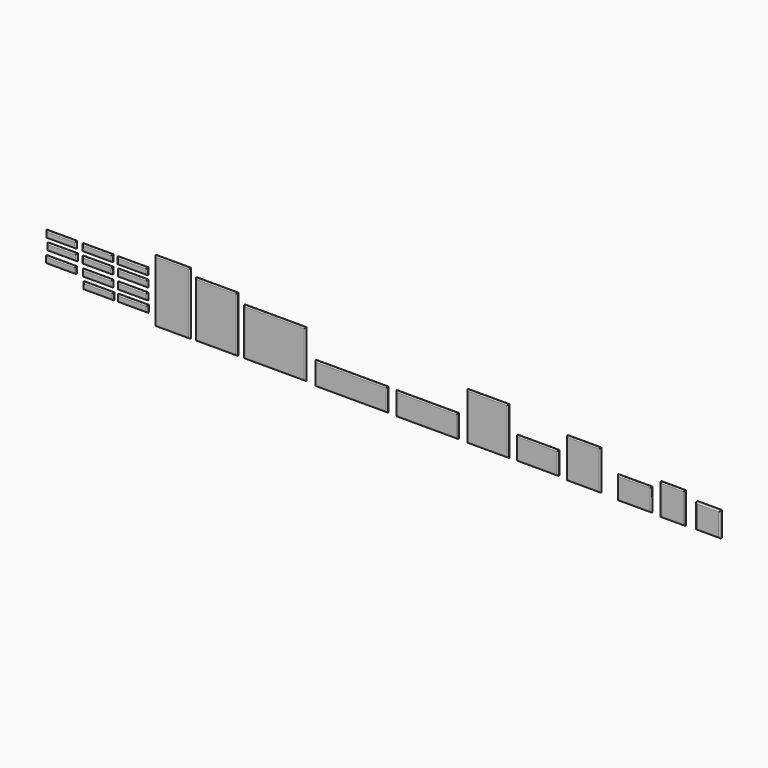
from build123d import *

# Parameters (mm, degrees)
F0_W           = 123
F0_H           = 28
F1_DEPTH       = 10
F2_T           = -2.5
F2_2_T         = -2.5
F2_3_T         = -2.5
F2_4_T         = -2.5
F2_5_T         = -2.5
F2_6_T         = -2.5
F2_7_T         = -2.5
F2_8_T         = -2.5
F2_9_T         = -2.5
F2_10_T        = -2.5
F2_11_T        = -2.5
F3_W           = 144
F3_H           = 255
F4_DEPTH       = 10
F3_W_2         = 170
F3_H_2         = 227
F3_W_3         = 253
F3_H_3         = 193
F3_W_4         = 296
F3_H_4         = 93
F3_W_5         = 139
F3_H_5         = 162
F3_W_6         = 100
F3_H_6         = 128
F3_H_7         = 100
F5_T           = -2.5
F5_2_T         = -2.5
F5_3_T         = -2.5
F5_4_T         = -2.5
F5_5_T         = -2.5
F5_6_T         = -2.5
F5_7_T         = -2.5
F5_8_T         = -2.5
F5_9_T         = -2.5
F5_10_T        = -2.5
F5_11_T        = -2.5
F6_T1_DEPTH    = 169
F6_T3_DEPTH    = 280
F6_2_T1_DEPTH  = 252
F6_2_T3_DEPTH  = 195
F6_3_T1_DEPTH  = 278
F6_3_T3_DEPTH  = 218
F6_4_T1_DEPTH  = 118
F6_4_T3_DEPTH  = 321
F6_5_T1_DEPTH  = 278
F6_5_T3_DEPTH  = 118
F6_6_T1_DEPTH  = 195
F6_6_T3_DEPTH  = 218
F6_7_T1_DEPTH  = 195
F6_7_T3_DEPTH  = 118
F6_8_T1_DEPTH  = 164
F6_8_T3_DEPTH  = 187
F6_9_T1_DEPTH  = 164
F6_9_T3_DEPTH  = 118
F6_10_T1_DEPTH = 125
F6_10_T3_DEPTH = 153
F6_11_T1_DEPTH = 125
F6_11_T3_DEPTH = 125
F6_12_T1_DEPTH = 53
F6_12_T3_DEPTH = 148
F6_13_T1_DEPTH = 148
F6_13_T3_DEPTH = 53
F6_14_T1_DEPTH = 148
F6_14_T3_DEPTH = 53
F6_15_T1_DEPTH = 148
F6_15_T3_DEPTH = 53
F6_16_T1_DEPTH = 53
F6_16_T3_DEPTH = 148
F6_17_T1_DEPTH = 53
F6_17_T3_DEPTH = 148
F6_18_T1_DEPTH = 53
F6_18_T3_DEPTH = 148
F6_19_T1_DEPTH = 148
F6_19_T3_DEPTH = 53
F6_20_T1_DEPTH = 53
F6_20_T3_DEPTH = 148
F6_21_T1_DEPTH = 148
F6_21_T3_DEPTH = 53
F6_22_T1_DEPTH = 53
F6_22_T3_DEPTH = 148


# Not quite as in the source:
# - a fillet or chamfer that OpenCascade refuses, or shapes differently, is made with other operations: its cross-section is extruded or revolved along the edge and cut away or added


with BuildPart() as f1:
    # F0 (on Front) → F1 (new body)
    with BuildSketch(Plane.XZ):
        with Locations((-123.9206232131, 65.0202791235)):
            Rectangle(F0_W, F0_H)
    extrude(amount=F1_DEPTH)

    # F2
    f2_openings = [f1.faces().sort_by_distance(p)[0] for p in [
        (-123.920623, -5, 51.020279),
    ]]
    offset(amount=F2_T, openings=f2_openings)

    # F6#12: fillet of radius 5 on 8 edges, made by hand

    # F6_12_s2 → F6_12_t1 (cut)
    with BuildSketch(Plane.XY.offset(38.5202791235)):
        with BuildLine():
            ThreePointArc((-185.4206232131, -5), (-183.956157119, -8.5355339059), (-180.4206232131, -10))
            Line((-180.4206232131, -10), (-185.4206232131, -10))
            Line((-185.4206232131, -10), (-185.4206232131, -5))
        make_face()
        with BuildLine():
            ThreePointArc((-62.4206232131, -5), (-63.8850893071, -8.5355339059), (-67.4206232131, -10))
            Line((-67.4206232131, -10), (-62.4206232131, -10))
            Line((-62.4206232131, -10), (-62.4206232131, -5))
        make_face()
        with BuildLine():
            ThreePointArc((-185.4206232131, -5), (-183.956157119, -1.4644660941), (-180.4206232131, 0))
            Line((-180.4206232131, 0), (-185.4206232131, 0))
            Line((-185.4206232131, 0), (-185.4206232131, -5))
        make_face()
        with BuildLine():
            ThreePointArc((-62.4206232131, -5), (-63.8850893071, -1.4644660941), (-67.4206232131, 0))
            Line((-67.4206232131, 0), (-62.4206232131, 0))
            Line((-62.4206232131, 0), (-62.4206232131, -5))
        make_face()
    extrude(amount=F6_12_T1_DEPTH, mode=Mode.SUBTRACT)

    # F6_12_s4 → F6_12_t3 (cut)
    with BuildSketch(Plane.YZ.offset(-197.9206232131)):
        with BuildLine():
            ThreePointArc((-10, 56.0202791235), (-8.5355339059, 52.4847452176), (-5, 51.0202791235))
            Line((-5, 51.0202791235), (-10, 51.0202791235))
            Line((-10, 51.0202791235), (-10, 56.0202791235))
        make_face()
        with BuildLine():
            ThreePointArc((-5, 79.0202791235), (-8.5355339059, 77.5558130295), (-10, 74.0202791235))
            Line((-10, 74.0202791235), (-10, 79.0202791235))
            Line((-10, 79.0202791235), (-5, 79.0202791235))
        make_face()
        with BuildLine():
            ThreePointArc((0, 56.0202791235), (-1.4644660941, 52.4847452176), (-5, 51.0202791235))
            Line((-5, 51.0202791235), (0, 51.0202791235))
            Line((0, 51.0202791235), (0, 56.0202791235))
        make_face()
        with BuildLine():
            ThreePointArc((-5, 79.0202791235), (-1.4644660941, 77.5558130295), (0, 74.0202791235))
            Line((0, 74.0202791235), (0, 79.0202791235))
            Line((0, 79.0202791235), (-5, 79.0202791235))
        make_face()
    extrude(amount=F6_12_T3_DEPTH, mode=Mode.SUBTRACT)


with BuildPart() as f1b:
    # F0 (on Front) → F1, piece 2 (new body)
    with BuildSketch(Plane.XZ):
        with Locations((-123.1104342043, -25.217052117)):
            Rectangle(F0_W, F0_H)
    extrude(amount=F1_DEPTH)

    # F2#11
    f2_11_openings = [f1b.faces().sort_by_distance(p)[0] for p in [
        (-123.110434, -5, -39.217052),
    ]]
    offset(amount=F2_11_T, openings=f2_11_openings)

    # F6#16: fillet of radius 5 on 8 edges, made by hand

    # F6_16_s2 → F6_16_t1 (cut)
    with BuildSketch(Plane.XY.offset(-51.717052117)):
        with BuildLine():
            ThreePointArc((-61.6104342043, -5), (-63.0749002984, -8.5355339059), (-66.6104342043, -10))
            Line((-66.6104342043, -10), (-61.6104342043, -10))
            Line((-61.6104342043, -10), (-61.6104342043, -5))
        make_face()
        with BuildLine():
            ThreePointArc((-184.6104342043, -5), (-183.1459681103, -8.5355339059), (-179.6104342043, -10))
            Line((-179.6104342043, -10), (-184.6104342043, -10))
            Line((-184.6104342043, -10), (-184.6104342043, -5))
        make_face()
        with BuildLine():
            ThreePointArc((-61.6104342043, -5), (-63.0749002984, -1.4644660941), (-66.6104342043, 0))
            Line((-66.6104342043, 0), (-61.6104342043, 0))
            Line((-61.6104342043, 0), (-61.6104342043, -5))
        make_face()
        with BuildLine():
            ThreePointArc((-184.6104342043, -5), (-183.1459681103, -1.4644660941), (-179.6104342043, 0))
            Line((-179.6104342043, 0), (-184.6104342043, 0))
            Line((-184.6104342043, 0), (-184.6104342043, -5))
        make_face()
    extrude(amount=F6_16_T1_DEPTH, mode=Mode.SUBTRACT)

    # F6_16_s4 → F6_16_t3 (cut)
    with BuildSketch(Plane.YZ.offset(-197.1104342043)):
        with BuildLine():
            ThreePointArc((-5, -11.217052117), (-8.5355339059, -12.6815182111), (-10, -16.217052117))
            Line((-10, -16.217052117), (-10, -11.217052117))
            Line((-10, -11.217052117), (-5, -11.217052117))
        make_face()
        with BuildLine():
            ThreePointArc((-10, -34.217052117), (-8.5355339059, -37.7525860229), (-5, -39.217052117))
            Line((-5, -39.217052117), (-10, -39.217052117))
            Line((-10, -39.217052117), (-10, -34.217052117))
        make_face()
        with BuildLine():
            ThreePointArc((-5, -11.217052117), (-1.4644660941, -12.6815182111), (0, -16.217052117))
            Line((0, -16.217052117), (0, -11.217052117))
            Line((0, -11.217052117), (-5, -11.217052117))
        make_face()
        with BuildLine():
            ThreePointArc((0, -34.217052117), (-1.4644660941, -37.7525860229), (-5, -39.217052117))
            Line((-5, -39.217052117), (0, -39.217052117))
            Line((0, -39.217052117), (0, -34.217052117))
        make_face()
    extrude(amount=F6_16_T3_DEPTH, mode=Mode.SUBTRACT)


with BuildPart() as f1c:
    # F0 (on Front) → F1, piece 3 (new body)
    with BuildSketch(Plane.XZ):
        with Locations((-122.2762821019, -69.5036254227)):
            Rectangle(F0_W, F0_H)
    extrude(amount=F1_DEPTH)

    # F2#10
    f2_10_openings = [f1c.faces().sort_by_distance(p)[0] for p in [
        (-122.276282, -5, -83.503625),
    ]]
    offset(amount=F2_10_T, openings=f2_10_openings)

    # F6#15: fillet of radius 5 on 8 edges, made by hand

    # F6_15_s2 → F6_15_t1 (cut)
    with BuildSketch(Plane.YZ.offset(-196.2762821019)):
        with BuildLine():
            ThreePointArc((-5, -55.5036254227), (-8.5355339059, -56.9680915168), (-10, -60.5036254227))
            Line((-10, -60.5036254227), (-10, -55.5036254227))
            Line((-10, -55.5036254227), (-5, -55.5036254227))
        make_face()
        with BuildLine():
            ThreePointArc((-10, -78.5036254227), (-8.5355339059, -82.0391593286), (-5, -83.5036254227))
            Line((-5, -83.5036254227), (-10, -83.5036254227))
            Line((-10, -83.5036254227), (-10, -78.5036254227))
        make_face()
        with BuildLine():
            ThreePointArc((-5, -55.5036254227), (-1.4644660941, -56.9680915168), (0, -60.5036254227))
            Line((0, -60.5036254227), (0, -55.5036254227))
            Line((0, -55.5036254227), (-5, -55.5036254227))
        make_face()
        with BuildLine():
            ThreePointArc((0, -78.5036254227), (-1.4644660941, -82.0391593286), (-5, -83.5036254227))
            Line((-5, -83.5036254227), (0, -83.5036254227))
            Line((0, -83.5036254227), (0, -78.5036254227))
        make_face()
    extrude(amount=F6_15_T1_DEPTH, mode=Mode.SUBTRACT)

    # F6_15_s4 → F6_15_t3 (cut)
    with BuildSketch(Plane.XY.offset(-96.0036254227)):
        with BuildLine():
            ThreePointArc((-183.7762821019, -5), (-182.3118160078, -8.5355339059), (-178.7762821019, -10))
            Line((-178.7762821019, -10), (-183.7762821019, -10))
            Line((-183.7762821019, -10), (-183.7762821019, -5))
        make_face()
        with BuildLine():
            ThreePointArc((-60.7762821019, -5), (-62.2407481959, -8.5355339059), (-65.7762821019, -10))
            Line((-65.7762821019, -10), (-60.7762821019, -10))
            Line((-60.7762821019, -10), (-60.7762821019, -5))
        make_face()
        with BuildLine():
            ThreePointArc((-183.7762821019, -5), (-182.3118160078, -1.4644660941), (-178.7762821019, 0))
            Line((-178.7762821019, 0), (-183.7762821019, 0))
            Line((-183.7762821019, 0), (-183.7762821019, -5))
        make_face()
        with BuildLine():
            ThreePointArc((-60.7762821019, -5), (-62.2407481959, -1.4644660941), (-65.7762821019, 0))
            Line((-65.7762821019, 0), (-60.7762821019, 0))
            Line((-60.7762821019, 0), (-60.7762821019, -5))
        make_face()
    extrude(amount=F6_15_T3_DEPTH, mode=Mode.SUBTRACT)


with BuildPart() as f1d:
    # F0 (on Front) → F1, piece 4 (new body)
    with BuildSketch(Plane.XZ):
        with Locations((-267.2222574949, 65.6239078045)):
            Rectangle(F0_W, F0_H)
    extrude(amount=F1_DEPTH)

    # F2#4
    f2_4_openings = [f1d.faces().sort_by_distance(p)[0] for p in [
        (-267.222257, -5, 51.623908),
    ]]
    offset(amount=F2_4_T, openings=f2_4_openings)

    # F6#14: fillet of radius 5 on 8 edges, made by hand

    # F6_14_s2 → F6_14_t1 (cut)
    with BuildSketch(Plane.YZ.offset(-341.2222574949)):
        with BuildLine():
            ThreePointArc((-5, 79.6239078045), (-8.5355339059, 78.1594417104), (-10, 74.6239078045))
            Line((-10, 74.6239078045), (-10, 79.6239078045))
            Line((-10, 79.6239078045), (-5, 79.6239078045))
        make_face()
        with BuildLine():
            ThreePointArc((-10, 56.6239078045), (-8.5355339059, 53.0883738986), (-5, 51.6239078045))
            Line((-5, 51.6239078045), (-10, 51.6239078045))
            Line((-10, 51.6239078045), (-10, 56.6239078045))
        make_face()
        with BuildLine():
            ThreePointArc((-5, 79.6239078045), (-1.4644660941, 78.1594417104), (0, 74.6239078045))
            Line((0, 74.6239078045), (0, 79.6239078045))
            Line((0, 79.6239078045), (-5, 79.6239078045))
        make_face()
        with BuildLine():
            ThreePointArc((0, 56.6239078045), (-1.4644660941, 53.0883738986), (-5, 51.6239078045))
            Line((-5, 51.6239078045), (0, 51.6239078045))
            Line((0, 51.6239078045), (0, 56.6239078045))
        make_face()
    extrude(amount=F6_14_T1_DEPTH, mode=Mode.SUBTRACT)

    # F6_14_s4 → F6_14_t3 (cut)
    with BuildSketch(Plane.XY.offset(39.1239078045)):
        with BuildLine():
            ThreePointArc((-328.7222574949, -5), (-327.2577914009, -8.5355339059), (-323.7222574949, -10))
            Line((-323.7222574949, -10), (-328.7222574949, -10))
            Line((-328.7222574949, -10), (-328.7222574949, -5))
        make_face()
        with BuildLine():
            ThreePointArc((-205.7222574949, -5), (-207.186723589, -8.5355339059), (-210.7222574949, -10))
            Line((-210.7222574949, -10), (-205.7222574949, -10))
            Line((-205.7222574949, -10), (-205.7222574949, -5))
        make_face()
        with BuildLine():
            ThreePointArc((-328.7222574949, -5), (-327.2577914009, -1.4644660941), (-323.7222574949, 0))
            Line((-323.7222574949, 0), (-328.7222574949, 0))
            Line((-328.7222574949, 0), (-328.7222574949, -5))
        make_face()
        with BuildLine():
            ThreePointArc((-205.7222574949, -5), (-207.186723589, -1.4644660941), (-210.7222574949, 0))
            Line((-210.7222574949, 0), (-205.7222574949, 0))
            Line((-205.7222574949, 0), (-205.7222574949, -5))
        make_face()
    extrude(amount=F6_14_T3_DEPTH, mode=Mode.SUBTRACT)


with BuildPart() as f1e:
    # F0 (on Front) → F1, piece 5 (new body)
    with BuildSketch(Plane.XZ):
        with Locations((-123.2876462638, 21.4466401041)):
            Rectangle(F0_W, F0_H)
    extrude(amount=F1_DEPTH)

    # F2#2
    f2_2_openings = [f1e.faces().sort_by_distance(p)[0] for p in [
        (-123.287646, -5, 7.44664),
    ]]
    offset(amount=F2_2_T, openings=f2_2_openings)

    # F6#13: fillet of radius 5 on 8 edges, made by hand

    # F6_13_s2 → F6_13_t1 (cut)
    with BuildSketch(Plane.YZ.offset(-197.2876462638)):
        with BuildLine():
            ThreePointArc((-5, 35.4466401041), (-8.5355339059, 33.98217401), (-10, 30.4466401041))
            Line((-10, 30.4466401041), (-10, 35.4466401041))
            Line((-10, 35.4466401041), (-5, 35.4466401041))
        make_face()
        with BuildLine():
            ThreePointArc((-10, 12.4466401041), (-8.5355339059, 8.9111061981), (-5, 7.4466401041))
            Line((-5, 7.4466401041), (-10, 7.4466401041))
            Line((-10, 7.4466401041), (-10, 12.4466401041))
        make_face()
        with BuildLine():
            ThreePointArc((-5, 35.4466401041), (-1.4644660941, 33.98217401), (0, 30.4466401041))
            Line((0, 30.4466401041), (0, 35.4466401041))
            Line((0, 35.4466401041), (-5, 35.4466401041))
        make_face()
        with BuildLine():
            ThreePointArc((0, 12.4466401041), (-1.4644660941, 8.9111061981), (-5, 7.4466401041))
            Line((-5, 7.4466401041), (0, 7.4466401041))
            Line((0, 7.4466401041), (0, 12.4466401041))
        make_face()
    extrude(amount=F6_13_T1_DEPTH, mode=Mode.SUBTRACT)

    # F6_13_s4 → F6_13_t3 (cut)
    with BuildSketch(Plane.XY.offset(-5.0533598959)):
        with BuildLine():
            ThreePointArc((-184.7876462638, -5), (-183.3231801698, -8.5355339059), (-179.7876462638, -10))
            Line((-179.7876462638, -10), (-184.7876462638, -10))
            Line((-184.7876462638, -10), (-184.7876462638, -5))
        make_face()
        with BuildLine():
            ThreePointArc((-61.7876462638, -5), (-63.2521123579, -8.5355339059), (-66.7876462638, -10))
            Line((-66.7876462638, -10), (-61.7876462638, -10))
            Line((-61.7876462638, -10), (-61.7876462638, -5))
        make_face()
        with BuildLine():
            ThreePointArc((-184.7876462638, -5), (-183.3231801698, -1.4644660941), (-179.7876462638, 0))
            Line((-179.7876462638, 0), (-184.7876462638, 0))
            Line((-184.7876462638, 0), (-184.7876462638, -5))
        make_face()
        with BuildLine():
            ThreePointArc((-61.7876462638, -5), (-63.2521123579, -1.4644660941), (-66.7876462638, 0))
            Line((-66.7876462638, 0), (-61.7876462638, 0))
            Line((-61.7876462638, 0), (-61.7876462638, -5))
        make_face()
    extrude(amount=F6_13_T3_DEPTH, mode=Mode.SUBTRACT)


with BuildPart() as f1f:
    # F0 (on Front) → F1, piece 6 (new body)
    with BuildSketch(Plane.XZ):
        with Locations((-267.200274229, 20.9451825023)):
            Rectangle(F0_W, F0_H)
    extrude(amount=F1_DEPTH)

    # F2#9
    f2_9_openings = [f1f.faces().sort_by_distance(p)[0] for p in [
        (-267.200274, -5, 6.945183),
    ]]
    offset(amount=F2_9_T, openings=f2_9_openings)

    # F6#17: fillet of radius 5 on 8 edges, made by hand

    # F6_17_s2 → F6_17_t1 (cut)
    with BuildSketch(Plane.XY.offset(-5.5548174977)):
        with BuildLine():
            ThreePointArc((-205.700274229, -5), (-207.1647403231, -8.5355339059), (-210.700274229, -10))
            Line((-210.700274229, -10), (-205.700274229, -10))
            Line((-205.700274229, -10), (-205.700274229, -5))
        make_face()
        with BuildLine():
            ThreePointArc((-328.700274229, -5), (-327.235808135, -8.5355339059), (-323.700274229, -10))
            Line((-323.700274229, -10), (-328.700274229, -10))
            Line((-328.700274229, -10), (-328.700274229, -5))
        make_face()
        with BuildLine():
            ThreePointArc((-205.700274229, -5), (-207.1647403231, -1.4644660941), (-210.700274229, 0))
            Line((-210.700274229, 0), (-205.700274229, 0))
            Line((-205.700274229, 0), (-205.700274229, -5))
        make_face()
        with BuildLine():
            ThreePointArc((-328.700274229, -5), (-327.235808135, -1.4644660941), (-323.700274229, 0))
            Line((-323.700274229, 0), (-328.700274229, 0))
            Line((-328.700274229, 0), (-328.700274229, -5))
        make_face()
    extrude(amount=F6_17_T1_DEPTH, mode=Mode.SUBTRACT)

    # F6_17_s4 → F6_17_t3 (cut)
    with BuildSketch(Plane.YZ.offset(-341.200274229)):
        with BuildLine():
            ThreePointArc((-5, 34.9451825023), (-8.5355339059, 33.4807164082), (-10, 29.9451825023))
            Line((-10, 29.9451825023), (-10, 34.9451825023))
            Line((-10, 34.9451825023), (-5, 34.9451825023))
        make_face()
        with BuildLine():
            ThreePointArc((-10, 11.9451825023), (-8.5355339059, 8.4096485963), (-5, 6.9451825023))
            Line((-5, 6.9451825023), (-10, 6.9451825023))
            Line((-10, 6.9451825023), (-10, 11.9451825023))
        make_face()
        with BuildLine():
            ThreePointArc((-5, 34.9451825023), (-1.4644660941, 33.4807164082), (0, 29.9451825023))
            Line((0, 29.9451825023), (0, 34.9451825023))
            Line((0, 34.9451825023), (-5, 34.9451825023))
        make_face()
        with BuildLine():
            ThreePointArc((0, 11.9451825023), (-1.4644660941, 8.4096485963), (-5, 6.9451825023))
            Line((-5, 6.9451825023), (0, 6.9451825023))
            Line((0, 6.9451825023), (0, 11.9451825023))
        make_face()
    extrude(amount=F6_17_T3_DEPTH, mode=Mode.SUBTRACT)


with BuildPart() as f1g:
    # F0 (on Front) → F1, piece 7 (new body)
    with BuildSketch(Plane.XZ):
        with Locations((-415.5285229683, 65.9489542842)):
            Rectangle(F0_W, F0_H)
    extrude(amount=F1_DEPTH)

    # F2#5
    f2_5_openings = [f1g.faces().sort_by_distance(p)[0] for p in [
        (-415.528523, -5, 51.948954),
    ]]
    offset(amount=F2_5_T, openings=f2_5_openings)

    # F6#19: fillet of radius 5 on 8 edges, made by hand

    # F6_19_s2 → F6_19_t1 (cut)
    with BuildSketch(Plane.YZ.offset(-489.5285229683)):
        with BuildLine():
            ThreePointArc((-5, 79.9489542842), (-8.5355339059, 78.4844881901), (-10, 74.9489542842))
            Line((-10, 74.9489542842), (-10, 79.9489542842))
            Line((-10, 79.9489542842), (-5, 79.9489542842))
        make_face()
        with BuildLine():
            ThreePointArc((-10, 56.9489542842), (-8.5355339059, 53.4134203783), (-5, 51.9489542842))
            Line((-5, 51.9489542842), (-10, 51.9489542842))
            Line((-10, 51.9489542842), (-10, 56.9489542842))
        make_face()
        with BuildLine():
            ThreePointArc((-5, 79.9489542842), (-1.4644660941, 78.4844881901), (0, 74.9489542842))
            Line((0, 74.9489542842), (0, 79.9489542842))
            Line((0, 79.9489542842), (-5, 79.9489542842))
        make_face()
        with BuildLine():
            ThreePointArc((0, 56.9489542842), (-1.4644660941, 53.4134203783), (-5, 51.9489542842))
            Line((-5, 51.9489542842), (0, 51.9489542842))
            Line((0, 51.9489542842), (0, 56.9489542842))
        make_face()
    extrude(amount=F6_19_T1_DEPTH, mode=Mode.SUBTRACT)

    # F6_19_s4 → F6_19_t3 (cut)
    with BuildSketch(Plane.XY.offset(39.4489542842)):
        with BuildLine():
            ThreePointArc((-477.0285229683, -5), (-475.5640568742, -8.5355339059), (-472.0285229683, -10))
            Line((-472.0285229683, -10), (-477.0285229683, -10))
            Line((-477.0285229683, -10), (-477.0285229683, -5))
        make_face()
        with BuildLine():
            ThreePointArc((-354.0285229683, -5), (-355.4929890624, -8.5355339059), (-359.0285229683, -10))
            Line((-359.0285229683, -10), (-354.0285229683, -10))
            Line((-354.0285229683, -10), (-354.0285229683, -5))
        make_face()
        with BuildLine():
            ThreePointArc((-477.0285229683, -5), (-475.5640568742, -1.4644660941), (-472.0285229683, 0))
            Line((-472.0285229683, 0), (-477.0285229683, 0))
            Line((-477.0285229683, 0), (-477.0285229683, -5))
        make_face()
        with BuildLine():
            ThreePointArc((-354.0285229683, -5), (-355.4929890624, -1.4644660941), (-359.0285229683, 0))
            Line((-359.0285229683, 0), (-354.0285229683, 0))
            Line((-354.0285229683, 0), (-354.0285229683, -5))
        make_face()
    extrude(amount=F6_19_T3_DEPTH, mode=Mode.SUBTRACT)


with BuildPart() as f1h:
    # F0 (on Front) → F1, piece 8 (new body)
    with BuildSketch(Plane.XZ):
        with Locations((-411.7354323864, 21.8576700091)):
            Rectangle(F0_W, F0_H)
    extrude(amount=F1_DEPTH)

    # F2#3
    f2_3_openings = [f1h.faces().sort_by_distance(p)[0] for p in [
        (-411.735432, -5, 7.85767),
    ]]
    offset(amount=F2_3_T, openings=f2_3_openings)

    # F6#18: fillet of radius 5 on 8 edges, made by hand

    # F6_18_s2 → F6_18_t1 (cut)
    with BuildSketch(Plane.XY.offset(-4.6423299909)):
        with BuildLine():
            ThreePointArc((-350.2354323864, -5), (-351.6998984805, -8.5355339059), (-355.2354323864, -10))
            Line((-355.2354323864, -10), (-350.2354323864, -10))
            Line((-350.2354323864, -10), (-350.2354323864, -5))
        make_face()
        with BuildLine():
            ThreePointArc((-473.2354323864, -5), (-471.7709662923, -8.5355339059), (-468.2354323864, -10))
            Line((-468.2354323864, -10), (-473.2354323864, -10))
            Line((-473.2354323864, -10), (-473.2354323864, -5))
        make_face()
        with BuildLine():
            ThreePointArc((-350.2354323864, -5), (-351.6998984805, -1.4644660941), (-355.2354323864, 0))
            Line((-355.2354323864, 0), (-350.2354323864, 0))
            Line((-350.2354323864, 0), (-350.2354323864, -5))
        make_face()
        with BuildLine():
            ThreePointArc((-473.2354323864, -5), (-471.7709662923, -1.4644660941), (-468.2354323864, 0))
            Line((-468.2354323864, 0), (-473.2354323864, 0))
            Line((-473.2354323864, 0), (-473.2354323864, -5))
        make_face()
    extrude(amount=F6_18_T1_DEPTH, mode=Mode.SUBTRACT)

    # F6_18_s4 → F6_18_t3 (cut)
    with BuildSketch(Plane.YZ.offset(-485.7354323864)):
        with BuildLine():
            ThreePointArc((-5, 35.8576700091), (-8.5355339059, 34.3932039151), (-10, 30.8576700091))
            Line((-10, 30.8576700091), (-10, 35.8576700091))
            Line((-10, 35.8576700091), (-5, 35.8576700091))
        make_face()
        with BuildLine():
            ThreePointArc((-10, 12.8576700091), (-8.5355339059, 9.3221361032), (-5, 7.8576700091))
            Line((-5, 7.8576700091), (-10, 7.8576700091))
            Line((-10, 7.8576700091), (-10, 12.8576700091))
        make_face()
        with BuildLine():
            ThreePointArc((-5, 35.8576700091), (-1.4644660941, 34.3932039151), (0, 30.8576700091))
            Line((0, 30.8576700091), (0, 35.8576700091))
            Line((0, 35.8576700091), (-5, 35.8576700091))
        make_face()
        with BuildLine():
            ThreePointArc((0, 12.8576700091), (-1.4644660941, 9.3221361032), (-5, 7.8576700091))
            Line((-5, 7.8576700091), (0, 7.8576700091))
            Line((0, 7.8576700091), (0, 12.8576700091))
        make_face()
    extrude(amount=F6_18_T3_DEPTH, mode=Mode.SUBTRACT)


with BuildPart() as f1i:
    # F0 (on Front) → F1, piece 9 (new body)
    with BuildSketch(Plane.XZ):
        with Locations((-416.7087843418, -25.9238691404)):
            Rectangle(F0_W, F0_H)
    extrude(amount=F1_DEPTH)

    # F2#6
    f2_6_openings = [f1i.faces().sort_by_distance(p)[0] for p in [
        (-416.708784, -5, -39.923869),
    ]]
    offset(amount=F2_6_T, openings=f2_6_openings)

    # F6#20: fillet of radius 5 on 8 edges, made by hand

    # F6_20_s2 → F6_20_t1 (cut)
    with BuildSketch(Plane.XY.offset(-52.4238691404)):
        with BuildLine():
            ThreePointArc((-478.2087843418, -5), (-476.7443182477, -8.5355339059), (-473.2087843418, -10))
            Line((-473.2087843418, -10), (-478.2087843418, -10))
            Line((-478.2087843418, -10), (-478.2087843418, -5))
        make_face()
        with BuildLine():
            ThreePointArc((-355.2087843418, -5), (-356.6732504359, -8.5355339059), (-360.2087843418, -10))
            Line((-360.2087843418, -10), (-355.2087843418, -10))
            Line((-355.2087843418, -10), (-355.2087843418, -5))
        make_face()
        with BuildLine():
            ThreePointArc((-478.2087843418, -5), (-476.7443182477, -1.4644660941), (-473.2087843418, 0))
            Line((-473.2087843418, 0), (-478.2087843418, 0))
            Line((-478.2087843418, 0), (-478.2087843418, -5))
        make_face()
        with BuildLine():
            ThreePointArc((-355.2087843418, -5), (-356.6732504359, -1.4644660941), (-360.2087843418, 0))
            Line((-360.2087843418, 0), (-355.2087843418, 0))
            Line((-355.2087843418, 0), (-355.2087843418, -5))
        make_face()
    extrude(amount=F6_20_T1_DEPTH, mode=Mode.SUBTRACT)

    # F6_20_s4 → F6_20_t3 (cut)
    with BuildSketch(Plane.YZ.offset(-490.7087843418)):
        with BuildLine():
            ThreePointArc((-10, -34.9238691404), (-8.5355339059, -38.4594030464), (-5, -39.9238691404))
            Line((-5, -39.9238691404), (-10, -39.9238691404))
            Line((-10, -39.9238691404), (-10, -34.9238691404))
        make_face()
        with BuildLine():
            ThreePointArc((-5, -11.9238691404), (-8.5355339059, -13.3883352345), (-10, -16.9238691404))
            Line((-10, -16.9238691404), (-10, -11.9238691404))
            Line((-10, -11.9238691404), (-5, -11.9238691404))
        make_face()
        with BuildLine():
            ThreePointArc((0, -34.9238691404), (-1.4644660941, -38.4594030464), (-5, -39.9238691404))
            Line((-5, -39.9238691404), (0, -39.9238691404))
            Line((0, -39.9238691404), (0, -34.9238691404))
        make_face()
        with BuildLine():
            ThreePointArc((-5, -11.9238691404), (-1.4644660941, -13.3883352345), (0, -16.9238691404))
            Line((0, -16.9238691404), (0, -11.9238691404))
            Line((0, -11.9238691404), (-5, -11.9238691404))
        make_face()
    extrude(amount=F6_20_T3_DEPTH, mode=Mode.SUBTRACT)


with BuildPart() as f1j:
    # F0 (on Front) → F1, piece 10 (new body)
    with BuildSketch(Plane.XZ):
        with Locations((-263.1299664974, -70.2425591052)):
            Rectangle(F0_W, F0_H)
    extrude(amount=F1_DEPTH)

    # F2#7
    f2_7_openings = [f1j.faces().sort_by_distance(p)[0] for p in [
        (-263.129966, -5, -84.242559),
    ]]
    offset(amount=F2_7_T, openings=f2_7_openings)

    # F6#21: fillet of radius 5 on 8 edges, made by hand

    # F6_21_s2 → F6_21_t1 (cut)
    with BuildSketch(Plane.YZ.offset(-337.1299664974)):
        with BuildLine():
            ThreePointArc((-5, -56.2425591052), (-8.5355339059, -57.7070251992), (-10, -61.2425591052))
            Line((-10, -61.2425591052), (-10, -56.2425591052))
            Line((-10, -56.2425591052), (-5, -56.2425591052))
        make_face()
        with BuildLine():
            ThreePointArc((-10, -79.2425591052), (-8.5355339059, -82.7780930111), (-5, -84.2425591052))
            Line((-5, -84.2425591052), (-10, -84.2425591052))
            Line((-10, -84.2425591052), (-10, -79.2425591052))
        make_face()
        with BuildLine():
            ThreePointArc((-5, -56.2425591052), (-1.4644660941, -57.7070251992), (0, -61.2425591052))
            Line((0, -61.2425591052), (0, -56.2425591052))
            Line((0, -56.2425591052), (-5, -56.2425591052))
        make_face()
        with BuildLine():
            ThreePointArc((0, -79.2425591052), (-1.4644660941, -82.7780930111), (-5, -84.2425591052))
            Line((-5, -84.2425591052), (0, -84.2425591052))
            Line((0, -84.2425591052), (0, -79.2425591052))
        make_face()
    extrude(amount=F6_21_T1_DEPTH, mode=Mode.SUBTRACT)

    # F6_21_s4 → F6_21_t3 (cut)
    with BuildSketch(Plane.XY.offset(-96.7425591052)):
        with BuildLine():
            ThreePointArc((-324.6299664974, -5), (-323.1655004034, -8.5355339059), (-319.6299664974, -10))
            Line((-319.6299664974, -10), (-324.6299664974, -10))
            Line((-324.6299664974, -10), (-324.6299664974, -5))
        make_face()
        with BuildLine():
            ThreePointArc((-201.6299664974, -5), (-203.0944325915, -8.5355339059), (-206.6299664974, -10))
            Line((-206.6299664974, -10), (-201.6299664974, -10))
            Line((-201.6299664974, -10), (-201.6299664974, -5))
        make_face()
        with BuildLine():
            ThreePointArc((-324.6299664974, -5), (-323.1655004034, -1.4644660941), (-319.6299664974, 0))
            Line((-319.6299664974, 0), (-324.6299664974, 0))
            Line((-324.6299664974, 0), (-324.6299664974, -5))
        make_face()
        with BuildLine():
            ThreePointArc((-201.6299664974, -5), (-203.0944325915, -1.4644660941), (-206.6299664974, 0))
            Line((-206.6299664974, 0), (-201.6299664974, 0))
            Line((-201.6299664974, 0), (-201.6299664974, -5))
        make_face()
    extrude(amount=F6_21_T3_DEPTH, mode=Mode.SUBTRACT)


with BuildPart() as f1k:
    # F0 (on Front) → F1, piece 11 (new body)
    with BuildSketch(Plane.XZ):
        with Locations((-266.2109156847, -25.3263549283)):
            Rectangle(F0_W, F0_H)
    extrude(amount=F1_DEPTH)

    # F2#8
    f2_8_openings = [f1k.faces().sort_by_distance(p)[0] for p in [
        (-266.210916, -5, -39.326355),
    ]]
    offset(amount=F2_8_T, openings=f2_8_openings)

    # F6#22: fillet of radius 5 on 8 edges, made by hand

    # F6_22_s2 → F6_22_t1 (cut)
    with BuildSketch(Plane.XY.offset(-51.8263549283)):
        with BuildLine():
            ThreePointArc((-327.7109156847, -5), (-326.2464495906, -8.5355339059), (-322.7109156847, -10))
            Line((-322.7109156847, -10), (-327.7109156847, -10))
            Line((-327.7109156847, -10), (-327.7109156847, -5))
        make_face()
        with BuildLine():
            ThreePointArc((-204.7109156847, -5), (-206.1753817788, -8.5355339059), (-209.7109156847, -10))
            Line((-209.7109156847, -10), (-204.7109156847, -10))
            Line((-204.7109156847, -10), (-204.7109156847, -5))
        make_face()
        with BuildLine():
            ThreePointArc((-327.7109156847, -5), (-326.2464495906, -1.4644660941), (-322.7109156847, 0))
            Line((-322.7109156847, 0), (-327.7109156847, 0))
            Line((-327.7109156847, 0), (-327.7109156847, -5))
        make_face()
        with BuildLine():
            ThreePointArc((-204.7109156847, -5), (-206.1753817788, -1.4644660941), (-209.7109156847, 0))
            Line((-209.7109156847, 0), (-204.7109156847, 0))
            Line((-204.7109156847, 0), (-204.7109156847, -5))
        make_face()
    extrude(amount=F6_22_T1_DEPTH, mode=Mode.SUBTRACT)

    # F6_22_s4 → F6_22_t3 (cut)
    with BuildSketch(Plane.YZ.offset(-340.2109156847)):
        with BuildLine():
            ThreePointArc((-10, -34.3263549283), (-8.5355339059, -37.8618888342), (-5, -39.3263549283))
            Line((-5, -39.3263549283), (-10, -39.3263549283))
            Line((-10, -39.3263549283), (-10, -34.3263549283))
        make_face()
        with BuildLine():
            ThreePointArc((-5, -11.3263549283), (-8.5355339059, -12.7908210224), (-10, -16.3263549283))
            Line((-10, -16.3263549283), (-10, -11.3263549283))
            Line((-10, -11.3263549283), (-5, -11.3263549283))
        make_face()
        with BuildLine():
            ThreePointArc((0, -34.3263549283), (-1.4644660941, -37.8618888342), (-5, -39.3263549283))
            Line((-5, -39.3263549283), (0, -39.3263549283))
            Line((0, -39.3263549283), (0, -34.3263549283))
        make_face()
        with BuildLine():
            ThreePointArc((-5, -11.3263549283), (-1.4644660941, -12.7908210224), (0, -16.3263549283))
            Line((0, -16.3263549283), (0, -11.3263549283))
            Line((0, -11.3263549283), (-5, -11.3263549283))
        make_face()
    extrude(amount=F6_22_T3_DEPTH, mode=Mode.SUBTRACT)


with BuildPart() as f4:
    # F3 (on Front) → F4 (new body)
    with BuildSketch(Plane.XZ):
        with Locations((40.7694758177, 6.803689003)):
            Rectangle(F3_W, F3_H)
    extrude(amount=F4_DEPTH)

    # F5
    f5_openings = [f4.faces().sort_by_distance(p)[0] for p in [
        (40.769476, -5, -120.696311),
    ]]
    offset(amount=F5_T, openings=f5_openings)

    # F6: fillet of radius 5 on 8 edges, made by hand

    # F6_s2 → F6_t1 (cut)
    with BuildSketch(Plane.YZ.offset(-43.7305241823)):
        with BuildLine():
            ThreePointArc((-10, -115.696310997), (-8.5355339059, -119.2318449029), (-5, -120.696310997))
            Line((-5, -120.696310997), (-10, -120.696310997))
            Line((-10, -120.696310997), (-10, -115.696310997))
        make_face()
        with BuildLine():
            ThreePointArc((-5, 134.303689003), (-8.5355339059, 132.8392229089), (-10, 129.303689003))
            Line((-10, 129.303689003), (-10, 134.303689003))
            Line((-10, 134.303689003), (-5, 134.303689003))
        make_face()
        with BuildLine():
            ThreePointArc((0, -115.696310997), (-1.4644660941, -119.2318449029), (-5, -120.696310997))
            Line((-5, -120.696310997), (0, -120.696310997))
            Line((0, -120.696310997), (0, -115.696310997))
        make_face()
        with BuildLine():
            ThreePointArc((-5, 134.303689003), (-1.4644660941, 132.8392229089), (0, 129.303689003))
            Line((0, 129.303689003), (0, 134.303689003))
            Line((0, 134.303689003), (-5, 134.303689003))
        make_face()
    extrude(amount=F6_T1_DEPTH, mode=Mode.SUBTRACT)

    # F6_s4 → F6_t3 (cut)
    with BuildSketch(Plane.XY.offset(-133.196310997)):
        with BuildLine():
            ThreePointArc((112.7694758177, -5), (111.3050097236, -8.5355339059), (107.7694758177, -10))
            Line((107.7694758177, -10), (112.7694758177, -10))
            Line((112.7694758177, -10), (112.7694758177, -5))
        make_face()
        with BuildLine():
            ThreePointArc((-31.2305241823, -5), (-29.7660580883, -8.5355339059), (-26.2305241823, -10))
            Line((-26.2305241823, -10), (-31.2305241823, -10))
            Line((-31.2305241823, -10), (-31.2305241823, -5))
        make_face()
        with BuildLine():
            ThreePointArc((112.7694758177, -5), (111.3050097236, -1.4644660941), (107.7694758177, 0))
            Line((107.7694758177, 0), (112.7694758177, 0))
            Line((112.7694758177, 0), (112.7694758177, -5))
        make_face()
        with BuildLine():
            ThreePointArc((-31.2305241823, -5), (-29.7660580883, -1.4644660941), (-26.2305241823, 0))
            Line((-26.2305241823, 0), (-31.2305241823, 0))
            Line((-31.2305241823, 0), (-31.2305241823, -5))
        make_face()
    extrude(amount=F6_T3_DEPTH, mode=Mode.SUBTRACT)


with BuildPart() as f4b:
    # F3 (on Front) → F4, piece 2 (new body)
    with BuildSketch(Plane.XZ):
        with Locations((220.5282962322, -5.895824194)):
            Rectangle(F3_W_2, F3_H_2)
    extrude(amount=F4_DEPTH)

    # F5#2
    f5_2_openings = [f4b.faces().sort_by_distance(p)[0] for p in [
        (220.528296, -5, -119.395824),
    ]]
    offset(amount=F5_2_T, openings=f5_2_openings)

    # F6#2: fillet of radius 5 on 8 edges, made by hand

    # F6_2_s2 → F6_2_t1 (cut)
    with BuildSketch(Plane.XY.offset(-131.895824194)):
        with BuildLine():
            ThreePointArc((305.5282962322, -5), (304.0638301382, -8.5355339059), (300.5282962322, -10))
            Line((300.5282962322, -10), (305.5282962322, -10))
            Line((305.5282962322, -10), (305.5282962322, -5))
        make_face()
        with BuildLine():
            ThreePointArc((135.5282962322, -5), (136.9927623263, -8.5355339059), (140.5282962322, -10))
            Line((140.5282962322, -10), (135.5282962322, -10))
            Line((135.5282962322, -10), (135.5282962322, -5))
        make_face()
        with BuildLine():
            ThreePointArc((305.5282962322, -5), (304.0638301382, -1.4644660941), (300.5282962322, 0))
            Line((300.5282962322, 0), (305.5282962322, 0))
            Line((305.5282962322, 0), (305.5282962322, -5))
        make_face()
        with BuildLine():
            ThreePointArc((135.5282962322, -5), (136.9927623263, -1.4644660941), (140.5282962322, 0))
            Line((140.5282962322, 0), (135.5282962322, 0))
            Line((135.5282962322, 0), (135.5282962322, -5))
        make_face()
    extrude(amount=F6_2_T1_DEPTH, mode=Mode.SUBTRACT)

    # F6_2_s4 → F6_2_t3 (cut)
    with BuildSketch(Plane.YZ.offset(123.0282962322)):
        with BuildLine():
            ThreePointArc((-5, 107.604175806), (-8.5355339059, 106.139709712), (-10, 102.604175806))
            Line((-10, 102.604175806), (-10, 107.604175806))
            Line((-10, 107.604175806), (-5, 107.604175806))
        make_face()
        with BuildLine():
            ThreePointArc((-10, -114.395824194), (-8.5355339059, -117.9313580999), (-5, -119.395824194))
            Line((-5, -119.395824194), (-10, -119.395824194))
            Line((-10, -119.395824194), (-10, -114.395824194))
        make_face()
        with BuildLine():
            ThreePointArc((-5, 107.604175806), (-1.4644660941, 106.139709712), (0, 102.604175806))
            Line((0, 102.604175806), (0, 107.604175806))
            Line((0, 107.604175806), (-5, 107.604175806))
        make_face()
        with BuildLine():
            ThreePointArc((0, -114.395824194), (-1.4644660941, -117.9313580999), (-5, -119.395824194))
            Line((-5, -119.395824194), (0, -119.395824194))
            Line((0, -119.395824194), (0, -114.395824194))
        make_face()
    extrude(amount=F6_2_T3_DEPTH, mode=Mode.SUBTRACT)


with BuildPart() as f4c:
    # F3 (on Front) → F4, piece 3 (new body)
    with BuildSketch(Plane.XZ):
        with Locations((458.9415385723, -22.597355783)):
            Rectangle(F3_W_3, F3_H_3)
    extrude(amount=F4_DEPTH)

    # F5#3
    f5_3_openings = [f4c.faces().sort_by_distance(p)[0] for p in [
        (458.941539, -5, -119.097356),
    ]]
    offset(amount=F5_3_T, openings=f5_3_openings)

    # F6#3: fillet of radius 5 on 8 edges, made by hand

    # F6_3_s2 → F6_3_t1 (cut)
    with BuildSketch(Plane.YZ.offset(319.9415385723)):
        with BuildLine():
            ThreePointArc((-5, 73.902644217), (-8.5355339059, 72.4381781229), (-10, 68.902644217))
            Line((-10, 68.902644217), (-10, 73.902644217))
            Line((-10, 73.902644217), (-5, 73.902644217))
        make_face()
        with BuildLine():
            ThreePointArc((-10, -114.097355783), (-8.5355339059, -117.6328896889), (-5, -119.097355783))
            Line((-5, -119.097355783), (-10, -119.097355783))
            Line((-10, -119.097355783), (-10, -114.097355783))
        make_face()
        with BuildLine():
            ThreePointArc((-5, 73.902644217), (-1.4644660941, 72.4381781229), (0, 68.902644217))
            Line((0, 68.902644217), (0, 73.902644217))
            Line((0, 73.902644217), (-5, 73.902644217))
        make_face()
        with BuildLine():
            ThreePointArc((0, -114.097355783), (-1.4644660941, -117.6328896889), (-5, -119.097355783))
            Line((-5, -119.097355783), (0, -119.097355783))
            Line((0, -119.097355783), (0, -114.097355783))
        make_face()
    extrude(amount=F6_3_T1_DEPTH, mode=Mode.SUBTRACT)

    # F6_3_s4 → F6_3_t3 (cut)
    with BuildSketch(Plane.XY.offset(-131.597355783)):
        with BuildLine():
            ThreePointArc((332.4415385723, -5), (333.9060046664, -8.5355339059), (337.4415385723, -10))
            Line((337.4415385723, -10), (332.4415385723, -10))
            Line((332.4415385723, -10), (332.4415385723, -5))
        make_face()
        with BuildLine():
            ThreePointArc((585.4415385723, -5), (583.9770724782, -8.5355339059), (580.4415385723, -10))
            Line((580.4415385723, -10), (585.4415385723, -10))
            Line((585.4415385723, -10), (585.4415385723, -5))
        make_face()
        with BuildLine():
            ThreePointArc((332.4415385723, -5), (333.9060046664, -1.4644660941), (337.4415385723, 0))
            Line((337.4415385723, 0), (332.4415385723, 0))
            Line((332.4415385723, 0), (332.4415385723, -5))
        make_face()
        with BuildLine():
            ThreePointArc((585.4415385723, -5), (583.9770724782, -1.4644660941), (580.4415385723, 0))
            Line((580.4415385723, 0), (585.4415385723, 0))
            Line((585.4415385723, 0), (585.4415385723, -5))
        make_face()
    extrude(amount=F6_3_T3_DEPTH, mode=Mode.SUBTRACT)


with BuildPart() as f4d:
    # F3 (on Front) → F4, piece 4 (new body)
    with BuildSketch(Plane.XZ):
        with Locations((771.81112957, -77.4734962583)):
            Rectangle(F3_W_4, F3_H_4)
    extrude(amount=F4_DEPTH)

    # F5#4
    f5_4_openings = [f4d.faces().sort_by_distance(p)[0] for p in [
        (771.81113, -5, -123.973496),
    ]]
    offset(amount=F5_4_T, openings=f5_4_openings)

    # F6#4: fillet of radius 5 on 8 edges, made by hand

    # F6_4_s2 → F6_4_t1 (cut)
    with BuildSketch(Plane.XY.offset(-136.4734962583)):
        with BuildLine():
            ThreePointArc((919.81112957, -5), (918.3466634759, -8.5355339059), (914.81112957, -10))
            Line((914.81112957, -10), (919.81112957, -10))
            Line((919.81112957, -10), (919.81112957, -5))
        make_face()
        with BuildLine():
            ThreePointArc((623.81112957, -5), (625.2755956641, -8.5355339059), (628.81112957, -10))
            Line((628.81112957, -10), (623.81112957, -10))
            Line((623.81112957, -10), (623.81112957, -5))
        make_face()
        with BuildLine():
            ThreePointArc((919.81112957, -5), (918.3466634759, -1.4644660941), (914.81112957, 0))
            Line((914.81112957, 0), (919.81112957, 0))
            Line((919.81112957, 0), (919.81112957, -5))
        make_face()
        with BuildLine():
            ThreePointArc((623.81112957, -5), (625.2755956641, -1.4644660941), (628.81112957, 0))
            Line((628.81112957, 0), (623.81112957, 0))
            Line((623.81112957, 0), (623.81112957, -5))
        make_face()
    extrude(amount=F6_4_T1_DEPTH, mode=Mode.SUBTRACT)

    # F6_4_s4 → F6_4_t3 (cut)
    with BuildSketch(Plane.YZ.offset(611.31112957)):
        with BuildLine():
            ThreePointArc((-5, -30.9734962583), (-8.5355339059, -32.4379623523), (-10, -35.9734962583))
            Line((-10, -35.9734962583), (-10, -30.9734962583))
            Line((-10, -30.9734962583), (-5, -30.9734962583))
        make_face()
        with BuildLine():
            ThreePointArc((-10, -118.9734962583), (-8.5355339059, -122.5090301642), (-5, -123.9734962583))
            Line((-5, -123.9734962583), (-10, -123.9734962583))
            Line((-10, -123.9734962583), (-10, -118.9734962583))
        make_face()
        with BuildLine():
            ThreePointArc((-5, -30.9734962583), (-1.4644660941, -32.4379623523), (0, -35.9734962583))
            Line((0, -35.9734962583), (0, -30.9734962583))
            Line((0, -30.9734962583), (-5, -30.9734962583))
        make_face()
        with BuildLine():
            ThreePointArc((0, -118.9734962583), (-1.4644660941, -122.5090301642), (-5, -123.9734962583))
            Line((-5, -123.9734962583), (0, -123.9734962583))
            Line((0, -123.9734962583), (0, -118.9734962583))
        make_face()
    extrude(amount=F6_4_T3_DEPTH, mode=Mode.SUBTRACT)


with BuildPart() as f4e:
    # F3 (on Front) → F4, piece 5 (new body)
    with BuildSketch(Plane.XZ):
        with Locations((1081.6999778748, -78.9979163706)):
            Rectangle(F3_W_3, F3_H_4)
    extrude(amount=F4_DEPTH)

    # F5#5
    f5_5_openings = [f4e.faces().sort_by_distance(p)[0] for p in [
        (1081.699978, -5, -125.497916),
    ]]
    offset(amount=F5_5_T, openings=f5_5_openings)

    # F6#5: fillet of radius 5 on 8 edges, made by hand

    # F6_5_s2 → F6_5_t1 (cut)
    with BuildSketch(Plane.YZ.offset(942.6999778748)):
        with BuildLine():
            ThreePointArc((-5, -32.4979163706), (-8.5355339059, -33.9623824647), (-10, -37.4979163706))
            Line((-10, -37.4979163706), (-10, -32.4979163706))
            Line((-10, -32.4979163706), (-5, -32.4979163706))
        make_face()
        with BuildLine():
            ThreePointArc((-10, -120.4979163706), (-8.5355339059, -124.0334502766), (-5, -125.4979163706))
            Line((-5, -125.4979163706), (-10, -125.4979163706))
            Line((-10, -125.4979163706), (-10, -120.4979163706))
        make_face()
        with BuildLine():
            ThreePointArc((-5, -32.4979163706), (-1.4644660941, -33.9623824647), (0, -37.4979163706))
            Line((0, -37.4979163706), (0, -32.4979163706))
            Line((0, -32.4979163706), (-5, -32.4979163706))
        make_face()
        with BuildLine():
            ThreePointArc((0, -120.4979163706), (-1.4644660941, -124.0334502766), (-5, -125.4979163706))
            Line((-5, -125.4979163706), (0, -125.4979163706))
            Line((0, -125.4979163706), (0, -120.4979163706))
        make_face()
    extrude(amount=F6_5_T1_DEPTH, mode=Mode.SUBTRACT)

    # F6_5_s4 → F6_5_t3 (cut)
    with BuildSketch(Plane.XY.offset(-137.9979163706)):
        with BuildLine():
            ThreePointArc((955.1999778748, -5), (956.6644439688, -8.5355339059), (960.1999778748, -10))
            Line((960.1999778748, -10), (955.1999778748, -10))
            Line((955.1999778748, -10), (955.1999778748, -5))
        make_face()
        with BuildLine():
            ThreePointArc((1208.1999778748, -5), (1206.7355117807, -8.5355339059), (1203.1999778748, -10))
            Line((1203.1999778748, -10), (1208.1999778748, -10))
            Line((1208.1999778748, -10), (1208.1999778748, -5))
        make_face()
        with BuildLine():
            ThreePointArc((955.1999778748, -5), (956.6644439688, -1.4644660941), (960.1999778748, 0))
            Line((960.1999778748, 0), (955.1999778748, 0))
            Line((955.1999778748, 0), (955.1999778748, -5))
        make_face()
        with BuildLine():
            ThreePointArc((1208.1999778748, -5), (1206.7355117807, -1.4644660941), (1203.1999778748, 0))
            Line((1203.1999778748, 0), (1208.1999778748, 0))
            Line((1208.1999778748, 0), (1208.1999778748, -5))
        make_face()
    extrude(amount=F6_5_T3_DEPTH, mode=Mode.SUBTRACT)


with BuildPart() as f4f:
    # F3 (on Front) → F4, piece 6 (new body)
    with BuildSketch(Plane.XZ):
        with Locations((1330.2235984802, -29.8191215992)):
            Rectangle(F3_W_2, F3_H_3)
    extrude(amount=F4_DEPTH)

    # F5#6
    f5_6_openings = [f4f.faces().sort_by_distance(p)[0] for p in [
        (1330.223598, -5, -126.319122),
    ]]
    offset(amount=F5_6_T, openings=f5_6_openings)

    # F6#6: fillet of radius 5 on 8 edges, made by hand

    # F6_6_s2 → F6_6_t1 (cut)
    with BuildSketch(Plane.YZ.offset(1232.7235984802)):
        with BuildLine():
            ThreePointArc((-5, 66.6808784008), (-8.5355339059, 65.2164123067), (-10, 61.6808784008))
            Line((-10, 61.6808784008), (-10, 66.6808784008))
            Line((-10, 66.6808784008), (-5, 66.6808784008))
        make_face()
        with BuildLine():
            ThreePointArc((-10, -121.3191215992), (-8.5355339059, -124.8546555051), (-5, -126.3191215992))
            Line((-5, -126.3191215992), (-10, -126.3191215992))
            Line((-10, -126.3191215992), (-10, -121.3191215992))
        make_face()
        with BuildLine():
            ThreePointArc((-5, 66.6808784008), (-1.4644660941, 65.2164123067), (0, 61.6808784008))
            Line((0, 61.6808784008), (0, 66.6808784008))
            Line((0, 66.6808784008), (-5, 66.6808784008))
        make_face()
        with BuildLine():
            ThreePointArc((0, -121.3191215992), (-1.4644660941, -124.8546555051), (-5, -126.3191215992))
            Line((-5, -126.3191215992), (0, -126.3191215992))
            Line((0, -126.3191215992), (0, -121.3191215992))
        make_face()
    extrude(amount=F6_6_T1_DEPTH, mode=Mode.SUBTRACT)

    # F6_6_s4 → F6_6_t3 (cut)
    with BuildSketch(Plane.XY.offset(-138.8191215992)):
        with BuildLine():
            ThreePointArc((1245.2235984802, -5), (1246.6880645743, -8.5355339059), (1250.2235984802, -10))
            Line((1250.2235984802, -10), (1245.2235984802, -10))
            Line((1245.2235984802, -10), (1245.2235984802, -5))
        make_face()
        with BuildLine():
            ThreePointArc((1415.2235984802, -5), (1413.7591323862, -8.5355339059), (1410.2235984802, -10))
            Line((1410.2235984802, -10), (1415.2235984802, -10))
            Line((1415.2235984802, -10), (1415.2235984802, -5))
        make_face()
        with BuildLine():
            ThreePointArc((1245.2235984802, -5), (1246.6880645743, -1.4644660941), (1250.2235984802, 0))
            Line((1250.2235984802, 0), (1245.2235984802, 0))
            Line((1245.2235984802, 0), (1245.2235984802, -5))
        make_face()
        with BuildLine():
            ThreePointArc((1415.2235984802, -5), (1413.7591323862, -1.4644660941), (1410.2235984802, 0))
            Line((1410.2235984802, 0), (1415.2235984802, 0))
            Line((1415.2235984802, 0), (1415.2235984802, -5))
        make_face()
    extrude(amount=F6_6_T3_DEPTH, mode=Mode.SUBTRACT)


with BuildPart() as f4g:
    # F3 (on Front) → F4, piece 7 (new body)
    with BuildSketch(Plane.XZ):
        with Locations((1533.9251375198, -78.5164710283)):
            Rectangle(F3_W_2, F3_H_4)
    extrude(amount=F4_DEPTH)

    # F5#7
    f5_7_openings = [f4g.faces().sort_by_distance(p)[0] for p in [
        (1533.925138, -5, -125.016471),
    ]]
    offset(amount=F5_7_T, openings=f5_7_openings)

    # F6#7: fillet of radius 5 on 8 edges, made by hand

    # F6_7_s2 → F6_7_t1 (cut)
    with BuildSketch(Plane.YZ.offset(1436.4251375198)):
        with BuildLine():
            ThreePointArc((-5, -32.0164710283), (-8.5355339059, -33.4809371224), (-10, -37.0164710283))
            Line((-10, -37.0164710283), (-10, -32.0164710283))
            Line((-10, -32.0164710283), (-5, -32.0164710283))
        make_face()
        with BuildLine():
            ThreePointArc((-10, -120.0164710283), (-8.5355339059, -123.5520049343), (-5, -125.0164710283))
            Line((-5, -125.0164710283), (-10, -125.0164710283))
            Line((-10, -125.0164710283), (-10, -120.0164710283))
        make_face()
        with BuildLine():
            ThreePointArc((-5, -32.0164710283), (-1.4644660941, -33.4809371224), (0, -37.0164710283))
            Line((0, -37.0164710283), (0, -32.0164710283))
            Line((0, -32.0164710283), (-5, -32.0164710283))
        make_face()
        with BuildLine():
            ThreePointArc((0, -120.0164710283), (-1.4644660941, -123.5520049343), (-5, -125.0164710283))
            Line((-5, -125.0164710283), (0, -125.0164710283))
            Line((0, -125.0164710283), (0, -120.0164710283))
        make_face()
    extrude(amount=F6_7_T1_DEPTH, mode=Mode.SUBTRACT)

    # F6_7_s4 → F6_7_t3 (cut)
    with BuildSketch(Plane.XY.offset(-137.5164710283)):
        with BuildLine():
            ThreePointArc((1448.9251375198, -5), (1450.3896036139, -8.5355339059), (1453.9251375198, -10))
            Line((1453.9251375198, -10), (1448.9251375198, -10))
            Line((1448.9251375198, -10), (1448.9251375198, -5))
        make_face()
        with BuildLine():
            ThreePointArc((1618.9251375198, -5), (1617.4606714258, -8.5355339059), (1613.9251375198, -10))
            Line((1613.9251375198, -10), (1618.9251375198, -10))
            Line((1618.9251375198, -10), (1618.9251375198, -5))
        make_face()
        with BuildLine():
            ThreePointArc((1448.9251375198, -5), (1450.3896036139, -1.4644660941), (1453.9251375198, 0))
            Line((1453.9251375198, 0), (1448.9251375198, 0))
            Line((1448.9251375198, 0), (1448.9251375198, -5))
        make_face()
        with BuildLine():
            ThreePointArc((1618.9251375198, -5), (1617.4606714258, -1.4644660941), (1613.9251375198, 0))
            Line((1613.9251375198, 0), (1618.9251375198, 0))
            Line((1618.9251375198, 0), (1618.9251375198, -5))
        make_face()
    extrude(amount=F6_7_T3_DEPTH, mode=Mode.SUBTRACT)


with BuildPart() as f4h:
    # F3 (on Front) → F4, piece 8 (new body)
    with BuildSketch(Plane.XZ):
        with Locations((1723.0415649414, -48.0206569135)):
            Rectangle(F3_W_5, F3_H_5)
    extrude(amount=F4_DEPTH)

    # F5#8
    f5_8_openings = [f4h.faces().sort_by_distance(p)[0] for p in [
        (1723.041565, -5, -129.020657),
    ]]
    offset(amount=F5_8_T, openings=f5_8_openings)

    # F6#8: fillet of radius 5 on 8 edges, made by hand

    # F6_8_s2 → F6_8_t1 (cut)
    with BuildSketch(Plane.YZ.offset(1641.0415649414)):
        with BuildLine():
            ThreePointArc((-5, 32.9793430865), (-8.5355339059, 31.5148769924), (-10, 27.9793430865))
            Line((-10, 27.9793430865), (-10, 32.9793430865))
            Line((-10, 32.9793430865), (-5, 32.9793430865))
        make_face()
        with BuildLine():
            ThreePointArc((-10, -124.0206569135), (-8.5355339059, -127.5561908195), (-5, -129.0206569135))
            Line((-5, -129.0206569135), (-10, -129.0206569135))
            Line((-10, -129.0206569135), (-10, -124.0206569135))
        make_face()
        with BuildLine():
            ThreePointArc((-5, 32.9793430865), (-1.4644660941, 31.5148769924), (0, 27.9793430865))
            Line((0, 27.9793430865), (0, 32.9793430865))
            Line((0, 32.9793430865), (-5, 32.9793430865))
        make_face()
        with BuildLine():
            ThreePointArc((0, -124.0206569135), (-1.4644660941, -127.5561908195), (-5, -129.0206569135))
            Line((-5, -129.0206569135), (0, -129.0206569135))
            Line((0, -129.0206569135), (0, -124.0206569135))
        make_face()
    extrude(amount=F6_8_T1_DEPTH, mode=Mode.SUBTRACT)

    # F6_8_s4 → F6_8_t3 (cut)
    with BuildSketch(Plane.XY.offset(-141.5206569135)):
        with BuildLine():
            ThreePointArc((1653.5415649414, -5), (1655.0060310355, -8.5355339059), (1658.5415649414, -10))
            Line((1658.5415649414, -10), (1653.5415649414, -10))
            Line((1653.5415649414, -10), (1653.5415649414, -5))
        make_face()
        with BuildLine():
            ThreePointArc((1792.5415649414, -5), (1791.0770988473, -8.5355339059), (1787.5415649414, -10))
            Line((1787.5415649414, -10), (1792.5415649414, -10))
            Line((1792.5415649414, -10), (1792.5415649414, -5))
        make_face()
        with BuildLine():
            ThreePointArc((1653.5415649414, -5), (1655.0060310355, -1.4644660941), (1658.5415649414, 0))
            Line((1658.5415649414, 0), (1653.5415649414, 0))
            Line((1653.5415649414, 0), (1653.5415649414, -5))
        make_face()
        with BuildLine():
            ThreePointArc((1792.5415649414, -5), (1791.0770988473, -1.4644660941), (1787.5415649414, 0))
            Line((1787.5415649414, 0), (1792.5415649414, 0))
            Line((1792.5415649414, 0), (1792.5415649414, -5))
        make_face()
    extrude(amount=F6_8_T3_DEPTH, mode=Mode.SUBTRACT)


with BuildPart() as f4i:
    # F3 (on Front) → F4, piece 9 (new body)
    with BuildSketch(Plane.XZ):
        with Locations((1931.1673336029, -86.621073246)):
            Rectangle(F3_W_5, F3_H_4)
    extrude(amount=F4_DEPTH)

    # F5#9
    f5_9_openings = [f4i.faces().sort_by_distance(p)[0] for p in [
        (1931.167334, -5, -133.121073),
    ]]
    offset(amount=F5_9_T, openings=f5_9_openings)

    # F6#9: fillet of radius 5 on 8 edges, made by hand

    # F6_9_s2 → F6_9_t1 (cut)
    with BuildSketch(Plane.YZ.offset(1849.1673336029)):
        with BuildLine():
            ThreePointArc((-5, -40.121073246), (-8.5355339059, -41.5855393401), (-10, -45.121073246))
            Line((-10, -45.121073246), (-10, -40.121073246))
            Line((-10, -40.121073246), (-5, -40.121073246))
        make_face()
        with BuildLine():
            ThreePointArc((-10, -128.121073246), (-8.5355339059, -131.6566071519), (-5, -133.121073246))
            Line((-5, -133.121073246), (-10, -133.121073246))
            Line((-10, -133.121073246), (-10, -128.121073246))
        make_face()
        with BuildLine():
            ThreePointArc((-5, -40.121073246), (-1.4644660941, -41.5855393401), (0, -45.121073246))
            Line((0, -45.121073246), (0, -40.121073246))
            Line((0, -40.121073246), (-5, -40.121073246))
        make_face()
        with BuildLine():
            ThreePointArc((0, -128.121073246), (-1.4644660941, -131.6566071519), (-5, -133.121073246))
            Line((-5, -133.121073246), (0, -133.121073246))
            Line((0, -133.121073246), (0, -128.121073246))
        make_face()
    extrude(amount=F6_9_T1_DEPTH, mode=Mode.SUBTRACT)

    # F6_9_s4 → F6_9_t3 (cut)
    with BuildSketch(Plane.XY.offset(-145.621073246)):
        with BuildLine():
            ThreePointArc((1861.6673336029, -5), (1863.131799697, -8.5355339059), (1866.6673336029, -10))
            Line((1866.6673336029, -10), (1861.6673336029, -10))
            Line((1861.6673336029, -10), (1861.6673336029, -5))
        make_face()
        with BuildLine():
            ThreePointArc((2000.6673336029, -5), (1999.2028675088, -8.5355339059), (1995.6673336029, -10))
            Line((1995.6673336029, -10), (2000.6673336029, -10))
            Line((2000.6673336029, -10), (2000.6673336029, -5))
        make_face()
        with BuildLine():
            ThreePointArc((1861.6673336029, -5), (1863.131799697, -1.4644660941), (1866.6673336029, 0))
            Line((1866.6673336029, 0), (1861.6673336029, 0))
            Line((1861.6673336029, 0), (1861.6673336029, -5))
        make_face()
        with BuildLine():
            ThreePointArc((2000.6673336029, -5), (1999.2028675088, -1.4644660941), (1995.6673336029, 0))
            Line((1995.6673336029, 0), (2000.6673336029, 0))
            Line((2000.6673336029, 0), (2000.6673336029, -5))
        make_face()
    extrude(amount=F6_9_T3_DEPTH, mode=Mode.SUBTRACT)


with BuildPart() as f4j:
    # F3 (on Front) → F4, piece 10 (new body)
    with BuildSketch(Plane.XZ):
        with Locations((2086.7760658264, -72.4254043177)):
            Rectangle(F3_W_6, F3_H_6)
    extrude(amount=F4_DEPTH)

    # F5#10
    f5_10_openings = [f4j.faces().sort_by_distance(p)[0] for p in [
        (2086.776066, -5, -136.425404),
    ]]
    offset(amount=F5_10_T, openings=f5_10_openings)

    # F6#10: fillet of radius 5 on 8 edges, made by hand

    # F6_10_s2 → F6_10_t1 (cut)
    with BuildSketch(Plane.YZ.offset(2024.2760658264)):
        with BuildLine():
            ThreePointArc((-5, -8.4254043177), (-8.5355339059, -9.8898704117), (-10, -13.4254043177))
            Line((-10, -13.4254043177), (-10, -8.4254043177))
            Line((-10, -8.4254043177), (-5, -8.4254043177))
        make_face()
        with BuildLine():
            ThreePointArc((-10, -131.4254043177), (-8.5355339059, -134.9609382236), (-5, -136.4254043177))
            Line((-5, -136.4254043177), (-10, -136.4254043177))
            Line((-10, -136.4254043177), (-10, -131.4254043177))
        make_face()
        with BuildLine():
            ThreePointArc((-5, -8.4254043177), (-1.4644660941, -9.8898704117), (0, -13.4254043177))
            Line((0, -13.4254043177), (0, -8.4254043177))
            Line((0, -8.4254043177), (-5, -8.4254043177))
        make_face()
        with BuildLine():
            ThreePointArc((0, -131.4254043177), (-1.4644660941, -134.9609382236), (-5, -136.4254043177))
            Line((-5, -136.4254043177), (0, -136.4254043177))
            Line((0, -136.4254043177), (0, -131.4254043177))
        make_face()
    extrude(amount=F6_10_T1_DEPTH, mode=Mode.SUBTRACT)

    # F6_10_s4 → F6_10_t3 (cut)
    with BuildSketch(Plane.XY.offset(-148.9254043177)):
        with BuildLine():
            ThreePointArc((2036.7760658264, -5), (2038.2405319205, -8.5355339059), (2041.7760658264, -10))
            Line((2041.7760658264, -10), (2036.7760658264, -10))
            Line((2036.7760658264, -10), (2036.7760658264, -5))
        make_face()
        with BuildLine():
            ThreePointArc((2136.7760658264, -5), (2135.3115997323, -8.5355339059), (2131.7760658264, -10))
            Line((2131.7760658264, -10), (2136.7760658264, -10))
            Line((2136.7760658264, -10), (2136.7760658264, -5))
        make_face()
        with BuildLine():
            ThreePointArc((2036.7760658264, -5), (2038.2405319205, -1.4644660941), (2041.7760658264, 0))
            Line((2041.7760658264, 0), (2036.7760658264, 0))
            Line((2036.7760658264, 0), (2036.7760658264, -5))
        make_face()
        with BuildLine():
            ThreePointArc((2136.7760658264, -5), (2135.3115997323, -1.4644660941), (2131.7760658264, 0))
            Line((2131.7760658264, 0), (2136.7760658264, 0))
            Line((2136.7760658264, 0), (2136.7760658264, -5))
        make_face()
    extrude(amount=F6_10_T3_DEPTH, mode=Mode.SUBTRACT)


with BuildPart() as f4k:
    # F3 (on Front) → F4, piece 11 (new body)
    with BuildSketch(Plane.XZ):
        with Locations((2231.7815303802, -84.2666991055)):
            Rectangle(F3_W_6, F3_H_7)
    extrude(amount=F4_DEPTH)

    # F5#11
    f5_11_openings = [f4k.faces().sort_by_distance(p)[0] for p in [
        (2231.78153, -5, -134.266699),
    ]]
    offset(amount=F5_11_T, openings=f5_11_openings)

    # F6#11: fillet of radius 5 on 4 edges, made by hand

    # F6_11_s2 → F6_11_t1 (cut)
    with BuildSketch(Plane.YZ.offset(2169.2815303802)):
        with BuildLine():
            ThreePointArc((-5, -34.2666991055), (-8.5355339059, -35.7311651996), (-10, -39.2666991055))
            Line((-10, -39.2666991055), (-10, -34.2666991055))
            Line((-10, -34.2666991055), (-5, -34.2666991055))
        make_face()
        with BuildLine():
            ThreePointArc((-10, -129.2666991055), (-8.5355339059, -132.8022330114), (-5, -134.2666991055))
            Line((-5, -134.2666991055), (-10, -134.2666991055))
            Line((-10, -134.2666991055), (-10, -129.2666991055))
        make_face()
    extrude(amount=F6_11_T1_DEPTH, mode=Mode.SUBTRACT)

    # F6_11_s4 → F6_11_t3 (cut)
    with BuildSketch(Plane.XY.offset(-146.7666991055)):
        with BuildLine():
            ThreePointArc((2181.7815303802, -5), (2183.2459964743, -8.5355339059), (2186.7815303802, -10))
            Line((2186.7815303802, -10), (2181.7815303802, -10))
            Line((2181.7815303802, -10), (2181.7815303802, -5))
        make_face()
        with BuildLine():
            ThreePointArc((2281.7815303802, -5), (2280.3170642862, -8.5355339059), (2276.7815303802, -10))
            Line((2276.7815303802, -10), (2281.7815303802, -10))
            Line((2281.7815303802, -10), (2281.7815303802, -5))
        make_face()
    extrude(amount=F6_11_T3_DEPTH, mode=Mode.SUBTRACT)


solid = Compound([f1.part, f1b.part, f1c.part, f1d.part, f1e.part, f1f.part, f1g.part, f1h.part, f1i.part, f1j.part, f1k.part, f4.part, f4b.part, f4c.part, f4d.part, f4e.part, f4f.part, f4g.part, f4h.part, f4i.part, f4j.part, f4k.part])
